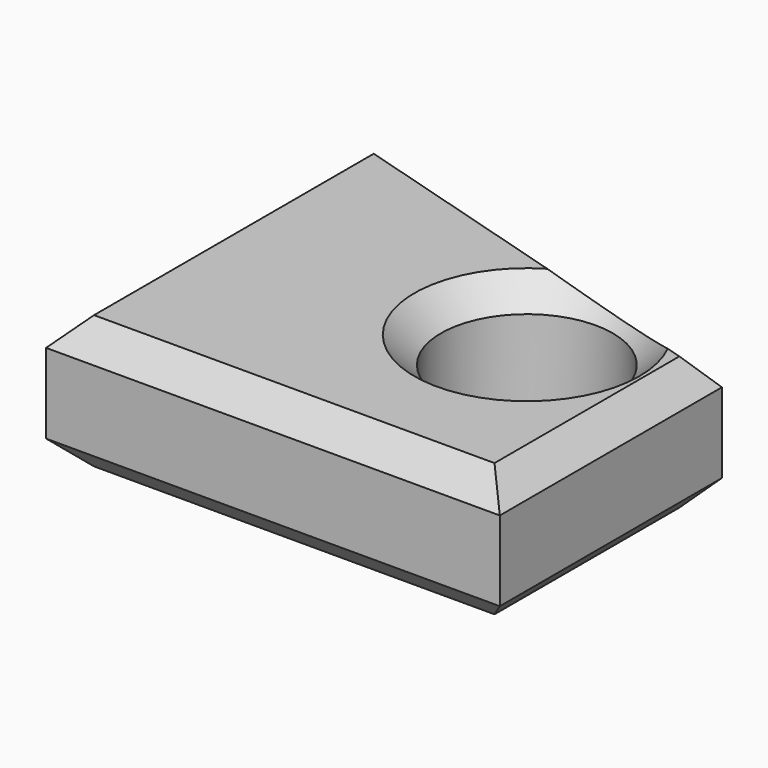
from build123d import *

# Parameters (mm, degrees)
F0_R        = 16.3870034363
F1_DEPTH    = 25.4
F2_T1_DEPTH = 116.4008158105
F2_T3_DEPTH = 104.7146316577
F2_T5_DEPTH = 112.6871608157
F2_T7_DEPTH = 79.0886539925
F3_T1_DEPTH = 116.4008158105
F3_T3_DEPTH = 104.7146316577
F3_T5_DEPTH = 112.6871608157
F3_T7_DEPTH = 79.0886539925


# Not quite as in the source:
# - a fillet or chamfer that OpenCascade refuses, or shapes differently, is made with other operations: its cross-section is extruded or revolved along the edge and cut away or added


with BuildPart() as f1:
    # F0 (on Top) → F1 (new body)
    with BuildSketch(Plane.XY):
        Polygon((27.1920096129, 8.1148929894), (-59.3668520451, 33.7408706546), (-59.3668520451, -44.8454618454), (27.1920096129, -44.8454618454), align=None)
        with Locations((0, -4.4133625925)):
            Circle(F0_R, mode=Mode.SUBTRACT)
    extrude(amount=F1_DEPTH)

    # F2: chamfer of 5.08 on 5 edges, made by hand

    # F2_s2 → F2_t1 (cut)
    with BuildSketch(Plane(origin=(35.3186398876, -10.4561758275, 0), x_dir=(0, 0, 1), z_dir=(-0.9588617319, 0.2838735267, 0))):
        Polygon((20.32, 15.5001520123), (25.4, 10.4201520123), (25.4, 15.5001520123), align=None)
    extrude(amount=F2_T1_DEPTH, mode=Mode.SUBTRACT)

    # F2_s4 → F2_t3 (cut)
    with BuildSketch(Plane.XZ.offset(-46.8050202334)):
        Polygon((-59.3668520451, 20.32), (-54.2868520451, 25.4), (-59.3668520451, 25.4), align=None)
    extrude(amount=F2_T3_DEPTH, mode=Mode.SUBTRACT)

    # F2_s6 → F2_t5 (cut)
    with BuildSketch(Plane.YZ.offset(-72.4310016239)):
        Polygon((-44.8454618454, 20.32), (-39.7654618454, 25.4), (-44.8454618454, 25.4), align=None)
    extrude(amount=F2_T5_DEPTH, mode=Mode.SUBTRACT)

    # F2_s8 → F2_t7 (cut)
    with BuildSketch(Plane.XZ.offset(-21.1790425683)):
        Polygon((27.1920096129, 20.32), (22.1120096129, 25.4), (27.1920096129, 25.4), align=None)
    extrude(amount=F2_T7_DEPTH, mode=Mode.SUBTRACT)

    # F2_s9 → F2_t10 (revolve, cut)
    with BuildSketch(Plane.XZ.offset(4.4133625925)):
        Polygon((16.3870034363, 20.32), (21.4670034363, 25.4), (16.3870034363, 25.4), align=None)
    revolve(axis=Axis((0, -4.4133625925, 25.4), (0, 0, 1)), mode=Mode.SUBTRACT)

    # F3: chamfer of 5.08 on 5 edges, made by hand

    # F3_s2 → F3_t1 (cut)
    with BuildSketch(Plane(origin=(35.3186398876, -10.4561758275, 0), x_dir=(0, 0, 1), z_dir=(-0.9588617319, 0.2838735267, 0))):
        Polygon((5.08, 15.5001520123), (0, 10.4201520123), (0, 15.5001520123), align=None)
    extrude(amount=F3_T1_DEPTH, mode=Mode.SUBTRACT)

    # F3_s4 → F3_t3 (cut)
    with BuildSketch(Plane.XZ.offset(-46.8050202334)):
        Polygon((-54.2868520451, 0), (-59.3668520451, 5.08), (-59.3668520451, 0), align=None)
    extrude(amount=F3_T3_DEPTH, mode=Mode.SUBTRACT)

    # F3_s6 → F3_t5 (cut)
    with BuildSketch(Plane.YZ.offset(-72.4310016239)):
        Polygon((-39.7654618454, 0), (-44.8454618454, 5.08), (-44.8454618454, 0), align=None)
    extrude(amount=F3_T5_DEPTH, mode=Mode.SUBTRACT)

    # F3_s8 → F3_t7 (cut)
    with BuildSketch(Plane.XZ.offset(-21.1790425683)):
        Polygon((22.1120096129, 0), (27.1920096129, 5.08), (27.1920096129, 0), align=None)
    extrude(amount=F3_T7_DEPTH, mode=Mode.SUBTRACT)

    # F3_s9 → F3_t10 (revolve, cut)
    with BuildSketch(Plane.XZ.offset(4.4133625925)):
        Polygon((21.4670034363, 0), (16.3870034363, 5.08), (16.3870034363, 0), align=None)
    revolve(axis=Axis((0, -4.4133625925, 0), (0, 0, 1)), mode=Mode.SUBTRACT)


solid = f1.part
